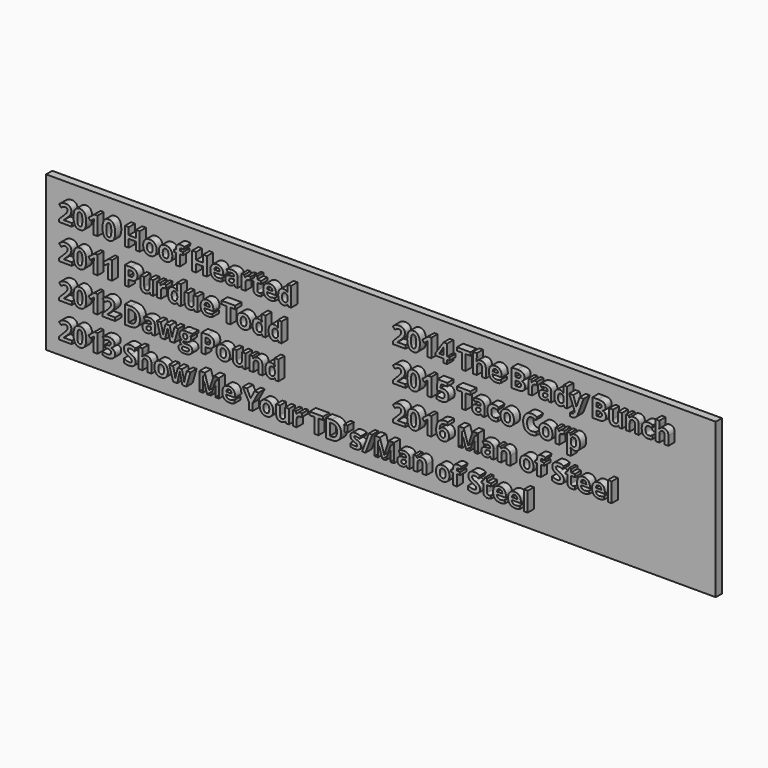
from build123d import *

# Parameters (mm, degrees)
F0_W         = 65
F0_H         = 30
F1_DEPTH     = 1.5
F2_TEXT_SIZE = 4.9237537548
F3_DEPTH     = 1.5
F4_TEXT_SIZE = 4.9237537548
F5_DEPTH     = 1.5


# Not quite as in the source:
# - Text() gives the source's letters only with a copy of the font that has no kerning and outlines rounded to 1/6400 em; it was checked with that copy


with BuildPart() as f1:
    # F0 (on Front) → F1 (new body)
    with BuildSketch(Plane.XZ):
        with Locations((32.5, 15)):
            Rectangle(F0_W, F0_H)
        with Locations((-32.5, 15)):
            Rectangle(F0_W, F0_H)
    extrude(amount=F1_DEPTH)

    # F2 (on face) → F3 (join)
    with BuildSketch(Plane.XZ.offset(1.5)):
        with Locations((3.319401294, 23.87712989)):
            Text('2014 The Brady Bunch', F2_TEXT_SIZE, font='Open Sans', font_style=FontStyle.BOLD, text_align=(TextAlign.LEFT, TextAlign.BOTTOM))
        with Locations((3.319401294, 17.1808247834)):
            Text('2015 Taco Corp', F2_TEXT_SIZE, font='Open Sans', font_style=FontStyle.BOLD, text_align=(TextAlign.LEFT, TextAlign.BOTTOM))
        with Locations((3.319401294, 10.4845196769)):
            Text('2016 Man of Steel', F2_TEXT_SIZE, font='Open Sans', font_style=FontStyle.BOLD, text_align=(TextAlign.LEFT, TextAlign.BOTTOM))
    extrude(amount=F3_DEPTH)

    # F4 (on face) → F5 (join)
    with BuildSketch(Plane.XZ.offset(1.5)):
        with Locations((-61.4609960732, 23.6730083508)):
            Text('2010 Hoof Hearted', F4_TEXT_SIZE, font='Open Sans', font_style=FontStyle.BOLD, text_align=(TextAlign.LEFT, TextAlign.BOTTOM))
        with Locations((-61.4609960732, 16.9767032442)):
            Text('2011 Purdue Todd', F4_TEXT_SIZE, font='Open Sans', font_style=FontStyle.BOLD, text_align=(TextAlign.LEFT, TextAlign.BOTTOM))
        with Locations((-61.4609960732, 10.2803981376)):
            Text('2012 Dawg Pound', F4_TEXT_SIZE, font='Open Sans', font_style=FontStyle.BOLD, text_align=(TextAlign.LEFT, TextAlign.BOTTOM))
        with Locations((-61.4609960732, 3.584093031)):
            Text("2013 Show Me Your TD's/Man of Steel", F4_TEXT_SIZE, font='Open Sans', font_style=FontStyle.BOLD, text_align=(TextAlign.LEFT, TextAlign.BOTTOM))
    extrude(amount=F5_DEPTH)


solid = f1.part
